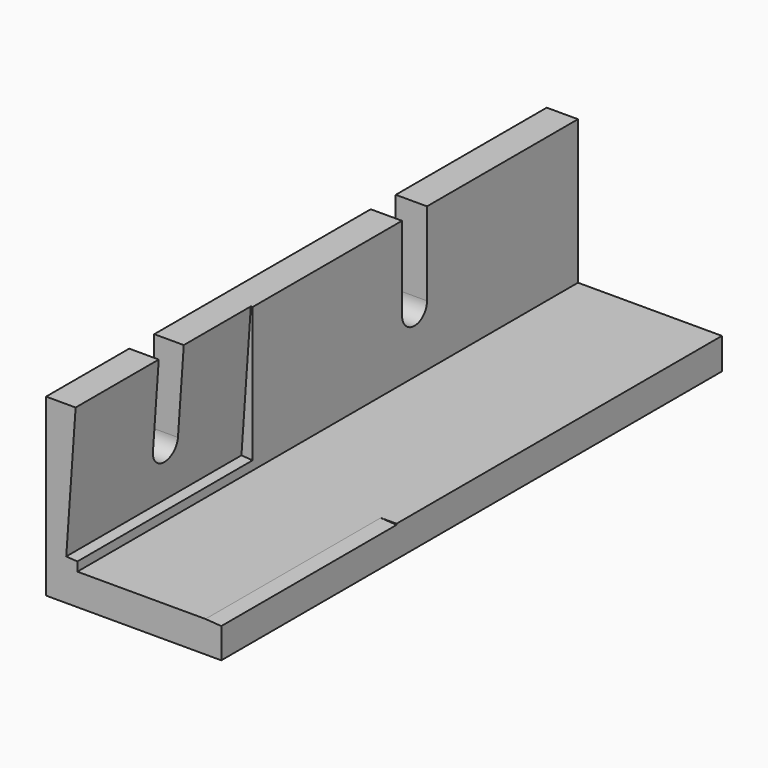
from build123d import *

# Parameters (mm, degrees)
F0_W     = 64.7085476667
F0_H     = 64.7085476667
F1_DEPTH = 127
F2_W     = 58.3585476667
F2_H     = 58.3585476667
F3_DEPTH = 127.001
F5_DEPTH = 44.45
F6_W     = 6.35
F6_H     = 24.0614805496
F7_DEPTH = 6.351
F9_DEPTH = 127.001


# Not quite as in the source:
# - a feature names something its author has since deleted; it is built from what else it names


with BuildPart() as f1:
    # F0 (on Front) → F1 (new body)
    with BuildSketch(Plane.XZ):
        with Locations((-1.2904843315, -7.374192588)):
            Rectangle(F0_W, F0_H)
    extrude(amount=-F1_DEPTH)

    # F2 (on face) → F3 (cut, through all)
    with BuildSketch(Plane(origin=(0, 127, 0), x_dir=(-1, 0, 0), z_dir=(0, 1, 0))):
        with Locations((-1.8845156685, -4.199192588)):
            Rectangle(F2_W, F2_H)
    extrude(amount=-F3_DEPTH, mode=Mode.SUBTRACT)

    # F4 (on face) → F5 (cut)
    with BuildSketch(Plane.XZ):
        Polygon((-27.2947581649, -31.5596693708), (-27.2947581649, 0.9186006957), (-29.554808952, -31.4016312239), align=None)
        Polygon((31.0637895018, -33.3784664214), (-1.2847486443, -33.3784664214), (31.0637895018, -35.6404965727), align=None)
    extrude(amount=-F5_DEPTH, mode=Mode.SUBTRACT)

    # F6 (on face) → F7 (cut, through all)
    with BuildSketch(Plane.YZ.offset(-27.2947581649)):
        with Locations((24.2636220248, 12.9493409705)):
            Rectangle(F6_W, F6_H)
        with BuildLine():
            Line((27.4386220248, -21.0581904151), (27.4386220248, 0.9186006957))
            Line((27.4386220248, 0.9186006957), (21.0886220248, 0.9186006957))
            Line((21.0886220248, 0.9186006957), (21.0886220248, -21.0581904151))
            ThreePointArc((21.0886220248, -21.0581904151), (24.2636220248, -24.2331904151), (27.4386220248, -21.0581904151))
        make_face()
        with BuildLine():
            Line((88.7001905876, 24.9800812453), (82.3501905876, 24.9800812453))
            Line((82.3501905876, 24.9800812453), (82.3501905876, -21.0581904151))
            ThreePointArc((82.3501905876, -21.0581904151), (85.5251905876, -24.2331904151), (88.7001905876, -21.0581904151))
            Line((88.7001905876, -21.0581904151), (88.7001905876, 24.9800812453))
        make_face()
    extrude(amount=-F7_DEPTH, mode=Mode.SUBTRACT)

    # F8 (on face) → F9 (cut, through all)
    with BuildSketch(Plane.XZ):
        Polygon((-27.2947581649, 0.9186006957), (-27.6504805517, -4.1684664214), (1.9152418351, -4.1684664214), (1.9152418351, 31.3519202173), (-33.6447581649, 31.3519202173), (-33.6447581649, 24.9800812453), (-27.2947581649, 24.9800812453), align=None)
        Polygon((-33.6447581649, 24.9800812453), (-33.6447581649, -4.1684664214), (-27.6504805517, -4.1684664214), (-27.2947581649, 0.9186006957), (-27.2947581649, 24.9800812453), align=None)
        Polygon((1.9152418351, -33.6022315546), (1.9152418351, -39.7284664214), (31.0637895018, -39.7284664214), (31.0637895018, -35.6404965727), align=None)
        Polygon((1.9152418351, -4.1684664214), (1.9152418351, -33.6022315546), (31.0637895018, -35.6404965727), (31.0637895018, 31.3519202173), (1.9152418351, 31.3519202173), align=None)
    extrude(amount=-F9_DEPTH, mode=Mode.SUBTRACT)


solid = f1.part
